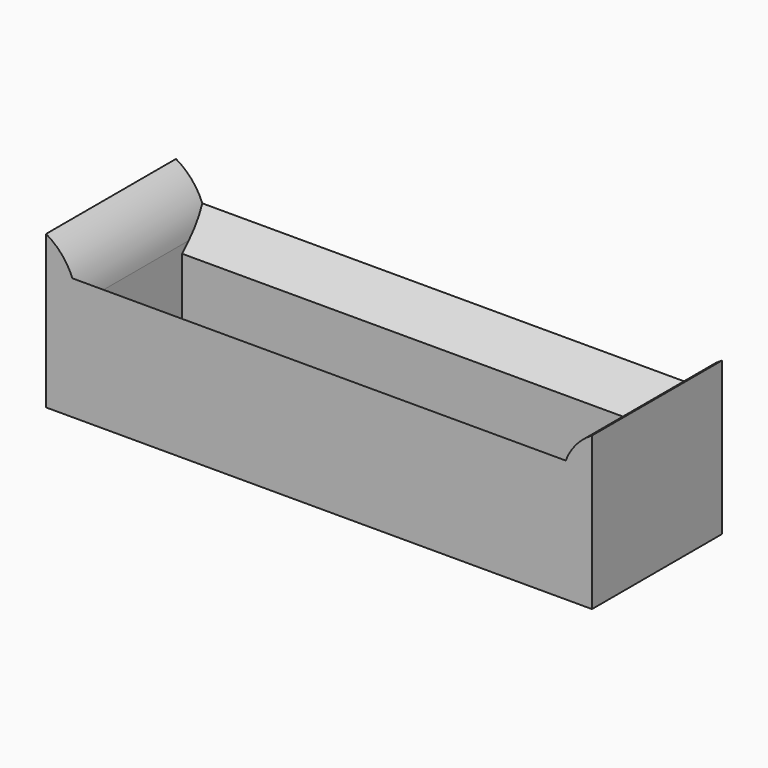
from build123d import *

# Parameters (mm, degrees)
F0_W         = 45.3698039055
F0_H         = 13.4970545769
F1_DEPTH     = 12.7
F2_T         = -2.54
F3_T1_DEPTH  = 40.2898039055
F4_T4_DEPTH  = 35.494099833
F4_T10_DEPTH = 35.494099833


# Not quite as in the source:
# - a fillet or chamfer that OpenCascade refuses, or shapes differently, is made with other operations: its cross-section is extruded or revolved along the edge and cut away or added


with BuildPart() as f1:
    # F0 (on Top) → F1 (new body)
    with BuildSketch(Plane.XY):
        with Locations((22.6849019527, -6.7485272884)):
            Rectangle(F0_W, F0_H)
    extrude(amount=F1_DEPTH)

    # F2
    f2_openings = [f1.faces().sort_by_distance(p)[0] for p in [
        (22.684902, -6.748527, 12.7),
    ]]
    offset(amount=F2_T, openings=f2_openings)

    # F3: chamfer of 5.08 on 2 edges, made by hand

    # F3_s2 → F3_t1 (cut)
    with BuildSketch(Plane.YZ.offset(2.54)):
        Polygon((-16.0370545769, 12.7), (-10.9570545769, 7.62), (-10.9570545769, 12.7), align=None)
        Polygon((2.54, 12.7), (-2.54, 7.62), (-2.54, 12.7), align=None)
    extrude(amount=F3_T1_DEPTH, mode=Mode.SUBTRACT)

    # F4: fillet of radius 5.08 on 2 edges, made by hand


with BuildPart() as f4_tool2:
    # F4_s3 → F4_t4 (new body)
    with BuildSketch(Plane.XZ.offset(24.4955772049)):
        with BuildLine():
            ThreePointArc((45.3698039055, 12.7), (43.5103948543, 10.8405909488), (42.8298039055, 8.3005909488))
            Line((42.8298039055, 8.3005909488), (42.8298039055, 12.7))
            Line((42.8298039055, 12.7), (45.3698039055, 12.7))
        make_face()
    extrude(amount=-F4_T4_DEPTH)

    split(bisect_by=Plane(origin=(0, -1.6685272884, -1.6685272884), x_dir=(1, 0, 0), z_dir=(0, 0.7071067812, 0.7071067812)), keep=Keep.TOP)

    split(bisect_by=Plane(origin=(0, -5.08, 5.08), x_dir=(1, 0, 0), z_dir=(0, -0.7071067812, 0.7071067812)), keep=Keep.TOP)


with BuildPart() as f1_1:
    add(f1.part)

    # F4_t1: cut F4_tool2
    add(f4_tool2.part, mode=Mode.SUBTRACT)


with BuildPart() as f4_tool8:
    # F4_s9 → F4_t10 (new body)
    with BuildSketch(Plane.XZ.offset(24.4955772049)):
        with BuildLine():
            ThreePointArc((2.54, 8.3005909488), (1.8594090512, 10.8405909488), (0, 12.7))
            Line((0, 12.7), (2.54, 12.7))
            Line((2.54, 12.7), (2.54, 8.3005909488))
        make_face()
    extrude(amount=-F4_T10_DEPTH)

    split(bisect_by=Plane(origin=(0, -1.6685272884, -1.6685272884), x_dir=(1, 0, 0), z_dir=(0, 0.7071067812, 0.7071067812)), keep=Keep.TOP)

    split(bisect_by=Plane(origin=(0, -5.08, 5.08), x_dir=(1, 0, 0), z_dir=(0, -0.7071067812, 0.7071067812)), keep=Keep.TOP)


with BuildPart() as f1_2:
    add(f1_1.part)

    # F4_t7: cut F4_tool8
    add(f4_tool8.part, mode=Mode.SUBTRACT)


solid = f1_2.part
